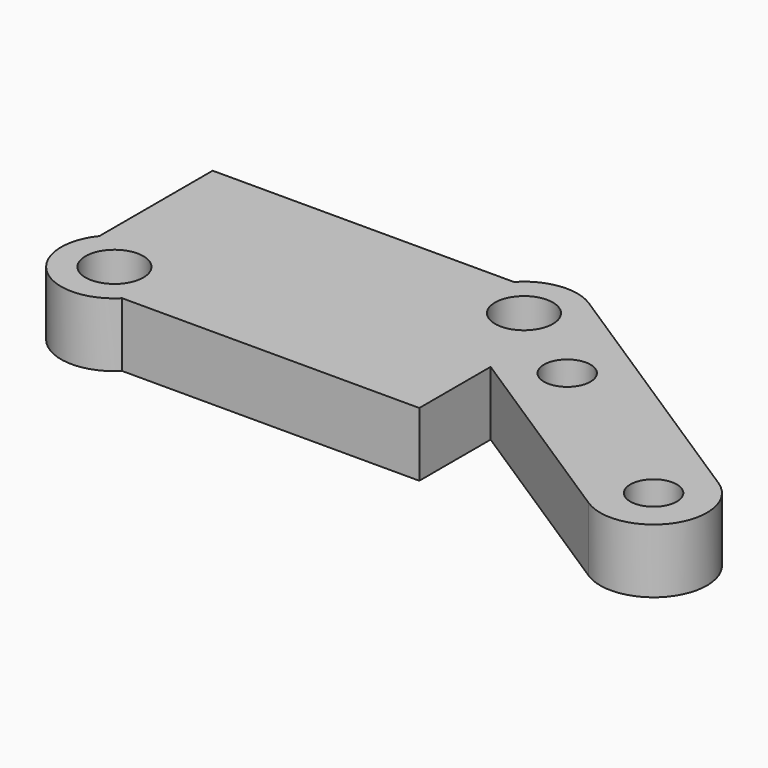
from build123d import *

# Parameters (mm, degrees)
F0_R     = 2.15265
F0_R_2   = 1.7272
F1_DEPTH = 4.7625


# Not quite as in the source:
# - a feature names something its author has since deleted; it is built from what else it names


with BuildPart() as f1:
    # F0 (on Top) → F1 (new body)
    with BuildSketch(Plane.XY):
        with BuildLine():
            Line((22.3912242158, 0), (0, 0))
            Line((0, 0), (0, -10.5219006149))
            ThreePointArc((0, -10.5219006149), (0.4570421145, -15.9607009606), (5.9126458296, -15.8))
            Line((5.9126458296, -15.8), (28, -15.8))
            Line((28, -15.8), (28, -9.1773860778))
            Line((28, -9.1773860778), (43.1353352142, -18.980828941))
            ThreePointArc((43.1353352142, -18.980828941), (48.6239542062, -17.8073662506), (47.4504915157, -12.3187472586))
            Line((47.4504915157, -12.3187472586), (27.4575781507, 0.6310408412))
            ThreePointArc((27.4575781507, 0.6310408412), (24.809461921, 1.2383180364), (22.3912242158, 0))
        make_face()
        with Locations((3.1, -13)):
            Circle(F0_R, mode=Mode.SUBTRACT)
        with Locations((45.2929133649, -15.6497880998)):
            Circle(F0_R_2, mode=Mode.SUBTRACT)
        with Locations((31.96875, -7.0194754969)):
            Circle(F0_R_2, mode=Mode.SUBTRACT)
        with Locations((25.3, -2.7)):
            Circle(F0_R, mode=Mode.SUBTRACT)
    extrude(amount=F1_DEPTH)


solid = f1.part
